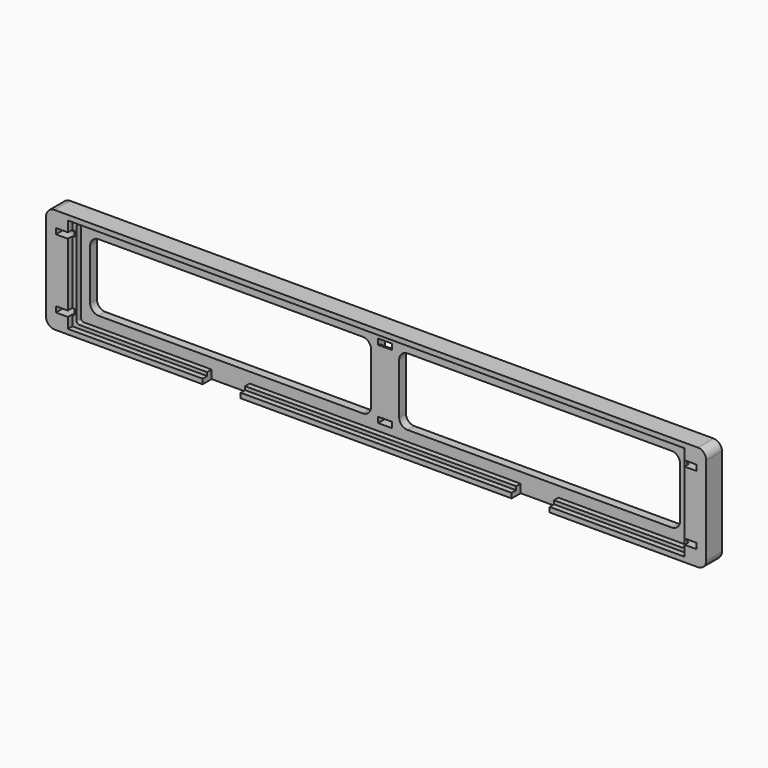
from build123d import *

# Parameters (mm, degrees)
F0_W        = 5
F0_H        = 2
F1_DEPTH    = 3
F2_W        = 5
F2_H        = 2
F3_DEPTH    = 4
F4_W        = 219.5
F4_H        = 34
F4_W_2      = 214.53166008
F4_H_2      = 28.9933998138
F5_DEPTH    = 2
F6_W        = 13.5
F6_H        = 4
F7_DEPTH    = 25
F8_T1_DEPTH = 5
F8_T3_DEPTH = 5
F8_T5_DEPTH = 5


# Not quite as in the source:
# - a fillet or chamfer that OpenCascade refuses, or shapes differently, is made with other operations: its cross-section is extruded or revolved along the edge and cut away or added
# - a feature names something its author has since deleted; it is built from what else it names


with BuildPart() as f1:
    # F0 (on Front) → F1 (new body)
    with BuildSketch(Plane.XZ):
        with BuildLine():
            ThreePointArc((117.5, 15.75), (116.6213203436, 17.8713203436), (114.5, 18.75))
            Line((114.5, 18.75), (-114.5, 18.75))
            ThreePointArc((-114.5, 18.75), (-116.6213203436, 17.8713203436), (-117.5, 15.75))
            Line((-117.5, 15.75), (-117.5, -15.75))
            ThreePointArc((-117.5, -15.75), (-116.6213203436, -17.8713203436), (-114.5, -18.75))
            Line((-114.5, -18.75), (114.5, -18.75))
            ThreePointArc((114.5, -18.75), (116.6213203436, -17.8713203436), (117.5, -15.75))
            Line((117.5, -15.75), (117.5, 15.75))
        make_face()
        with Locations((-111.5, -12.25)):
            Rectangle(F0_W, F0_H, mode=Mode.SUBTRACT)
        with Locations((0, -12.25)):
            Rectangle(F0_W, F0_H, mode=Mode.SUBTRACT)
        with Locations((111.5, -12.25)):
            Rectangle(F0_W, F0_H, mode=Mode.SUBTRACT)
        with BuildLine():
            Line((-102, 12), (-8, 12))
            ThreePointArc((-8, 12), (-5.8786796564, 11.1213203436), (-5, 9))
            Line((-5, 9), (-5, -9))
            ThreePointArc((-5, -9), (-5.8786796564, -11.1213203436), (-8, -12))
            Line((-8, -12), (-102, -12))
            ThreePointArc((-102, -12), (-104.1213203436, -11.1213203436), (-105, -9))
            Line((-105, -9), (-105, 9))
            ThreePointArc((-105, 9), (-104.1213203436, 11.1213203436), (-102, 12))
        make_face(mode=Mode.SUBTRACT)
        with Locations((-111.5, 12.25)):
            Rectangle(F0_W, F0_H, mode=Mode.SUBTRACT)
        with BuildLine():
            Line((8, 12), (102, 12))
            ThreePointArc((102, 12), (104.1213203436, 11.1213203436), (105, 9))
            Line((105, 9), (105, -9))
            ThreePointArc((105, -9), (104.1213203436, -11.1213203436), (102, -12))
            Line((102, -12), (8, -12))
            ThreePointArc((8, -12), (5.8786796564, -11.1213203436), (5, -9))
            Line((5, -9), (5, 9))
            ThreePointArc((5, 9), (5.8786796564, 11.1213203436), (8, 12))
        make_face(mode=Mode.SUBTRACT)
        with Locations((0, 12.25)):
            Rectangle(F0_W, F0_H, mode=Mode.SUBTRACT)
        with Locations((111.5, 12.25)):
            Rectangle(F0_W, F0_H, mode=Mode.SUBTRACT)
    extrude(amount=F1_DEPTH)

    # F2 (on face) → F3 (join)
    with BuildSketch(Plane.XZ.offset(3)):
        with BuildLine():
            Line((-114.5, -18.75), (114.5, -18.75))
            ThreePointArc((114.5, -18.75), (116.6213203436, -17.8713203436), (117.5, -15.75))
            Line((117.5, -15.75), (117.5, 15.75))
            ThreePointArc((117.5, 15.75), (116.6213203436, 17.8713203436), (114.5, 18.75))
            Line((114.5, 18.75), (-114.5, 18.75))
            ThreePointArc((-114.5, 18.75), (-116.6213203436, 17.8713203436), (-117.5, 15.75))
            Line((-117.5, 15.75), (-117.5, -15.75))
            ThreePointArc((-117.5, -15.75), (-116.6213203436, -17.8713203436), (-114.5, -18.75))
        make_face()
        with Locations((-111.5, -12.25)):
            Rectangle(F2_W, F2_H, mode=Mode.SUBTRACT)
        with Locations((111.5, -12.25)):
            Rectangle(F2_W, F2_H, mode=Mode.SUBTRACT)
        with BuildLine():
            Line((-107.25, 15.75), (107.25, 15.75))
            ThreePointArc((107.25, 15.75), (107.9571067812, 15.4571067812), (108.25, 14.75))
            Line((108.25, 14.75), (108.25, -14.75))
            ThreePointArc((108.25, -14.75), (107.9571067812, -15.4571067812), (107.25, -15.75))
            Line((107.25, -15.75), (-107.25, -15.75))
            ThreePointArc((-107.25, -15.75), (-107.9571067812, -15.4571067812), (-108.25, -14.75))
            Line((-108.25, -14.75), (-108.25, 14.75))
            ThreePointArc((-108.25, 14.75), (-107.9571067812, 15.4571067812), (-107.25, 15.75))
        make_face(mode=Mode.SUBTRACT)
        with Locations((-111.5, 12.25)):
            Rectangle(F2_W, F2_H, mode=Mode.SUBTRACT)
        with Locations((111.5, 12.25)):
            Rectangle(F2_W, F2_H, mode=Mode.SUBTRACT)
    extrude(amount=F3_DEPTH)

    # F4 (on face) → F5 (cut)
    with BuildSketch(Plane.XZ.offset(7)):
        Rectangle(F4_W, F4_H)
        Rectangle(F4_W_2, F4_H_2, mode=Mode.SUBTRACT)
    extrude(amount=-F5_DEPTH, mode=Mode.SUBTRACT)

    # F6 (on face) → F7 (cut)
    with BuildSketch(Plane(origin=(0, 0, -18.75), x_dir=(1, 0, 0), z_dir=(0, 0, -1))):
        with Locations((-55, 5)):
            Rectangle(F6_W, F6_H)
        with Locations((55, 5)):
            Rectangle(F6_W, F6_H)
    extrude(amount=-F7_DEPTH, mode=Mode.SUBTRACT)

    # F8: fillet of radius 3.5 on 6 edges, made by hand

    # F8_s2 → F8_t1 (cut)
    with BuildSketch(Plane.YZ.offset(-2.5)):
        with BuildLine():
            ThreePointArc((0, 7.7858983849), (-0.8542486889, 10.0771862323), (-3, 11.25))
            Line((-3, 11.25), (0, 11.25))
            Line((0, 11.25), (0, 7.7858983849))
        make_face()
        with BuildLine():
            ThreePointArc((0, -7.7858983849), (-0.8542486889, -10.0771862323), (-3, -11.25))
            Line((-3, -11.25), (0, -11.25))
            Line((0, -11.25), (0, -7.7858983849))
        make_face()
    extrude(amount=F8_T1_DEPTH, mode=Mode.SUBTRACT)

    # F8_s4 → F8_t3 (cut)
    with BuildSketch(Plane.YZ.offset(109)):
        with BuildLine():
            ThreePointArc((0, 7.75), (-1.0251262658, 10.2248737342), (-3.5, 11.25))
            Line((-3.5, 11.25), (0, 11.25))
            Line((0, 11.25), (0, 7.75))
        make_face()
        with BuildLine():
            ThreePointArc((0, -7.75), (-1.0251262658, -10.2248737342), (-3.5, -11.25))
            Line((-3.5, -11.25), (0, -11.25))
            Line((0, -11.25), (0, -7.75))
        make_face()
    extrude(amount=F8_T3_DEPTH, mode=Mode.SUBTRACT)

    # F8_s6 → F8_t5 (cut)
    with BuildSketch(Plane.YZ.offset(-114)):
        with BuildLine():
            ThreePointArc((0, -7.75), (-1.0251262658, -10.2248737342), (-3.5, -11.25))
            Line((-3.5, -11.25), (0, -11.25))
            Line((0, -11.25), (0, -7.75))
        make_face()
        with BuildLine():
            ThreePointArc((0, 7.75), (-1.0251262658, 10.2248737342), (-3.5, 11.25))
            Line((-3.5, 11.25), (0, 11.25))
            Line((0, 11.25), (0, 7.75))
        make_face()
    extrude(amount=F8_T5_DEPTH, mode=Mode.SUBTRACT)


solid = f1.part
